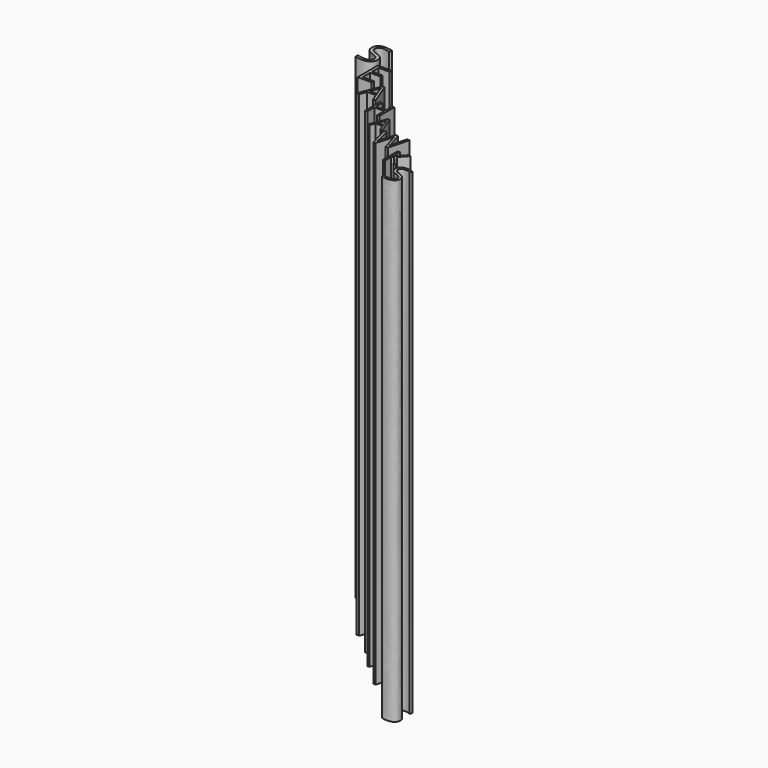
from build123d import *

# Parameters (mm, degrees)
F0_TEXT_SIZE   = 24.309888896
F0_TEXT_SIZE_2 = 22.5555565622
F0_TEXT_SIZE_3 = 19.2975418435
F0_TEXT_SIZE_4 = 16.7913734913
F0_TEXT_SIZE_5 = 15.2876600623
F0_TEXT_SIZE_6 = 18.0444369713
F0_TEXT_SIZE_7 = 16.5407442384
F0_TEXT_SIZE_8 = 20.3000174628
F1_DEPTH       = 304.8


# Not quite as in the source:
# - Text() gives the source's letters only with a copy of the font that has no kerning and outlines rounded to 1/6400 em; it was checked with that copy


with BuildPart() as f1:
    # F0 (on Top) → F1 (new body)
    with BuildSketch(Plane.XY):
        with Locations((-95.9964767098, 78.1324654818)):
            Text('S', F0_TEXT_SIZE, font='Open Sans', text_align=(TextAlign.LEFT, TextAlign.BOTTOM))
        with Locations((-82.2423973829, 61.892464757)):
            Text('E', F0_TEXT_SIZE_2, font='Open Sans', text_align=(TextAlign.LEFT, TextAlign.BOTTOM))
        with Locations((-69.5901398738, 47.9982346296)):
            Text('A', F0_TEXT_SIZE_3, font='Open Sans', text_align=(TextAlign.LEFT, TextAlign.BOTTOM))
        with Locations((-56.127089197, 35.9084457159)):
            Text('H', F0_TEXT_SIZE_4, font='Open Sans', text_align=(TextAlign.LEFT, TextAlign.BOTTOM))
        with Locations((-44.2891708857, 24.901330471)):
            Text('A', F0_TEXT_SIZE_5, font='Open Sans', text_align=(TextAlign.LEFT, TextAlign.BOTTOM))
        with Locations((-33.6236392953, 11.9093358517)):
            Text('W', F0_TEXT_SIZE_6, font='Open Sans', text_align=(TextAlign.LEFT, TextAlign.BOTTOM))
        with Locations((-15.9936604856, 0)):
            Text('K', F0_TEXT_SIZE_7, font='Open Sans', text_align=(TextAlign.LEFT, TextAlign.BOTTOM))
        with Locations((-4.7692148251, -14.6160125732)):
            Text('S', F0_TEXT_SIZE_8, font='Open Sans', text_align=(TextAlign.LEFT, TextAlign.BOTTOM))
    extrude(amount=F1_DEPTH)


solid = f1.part
